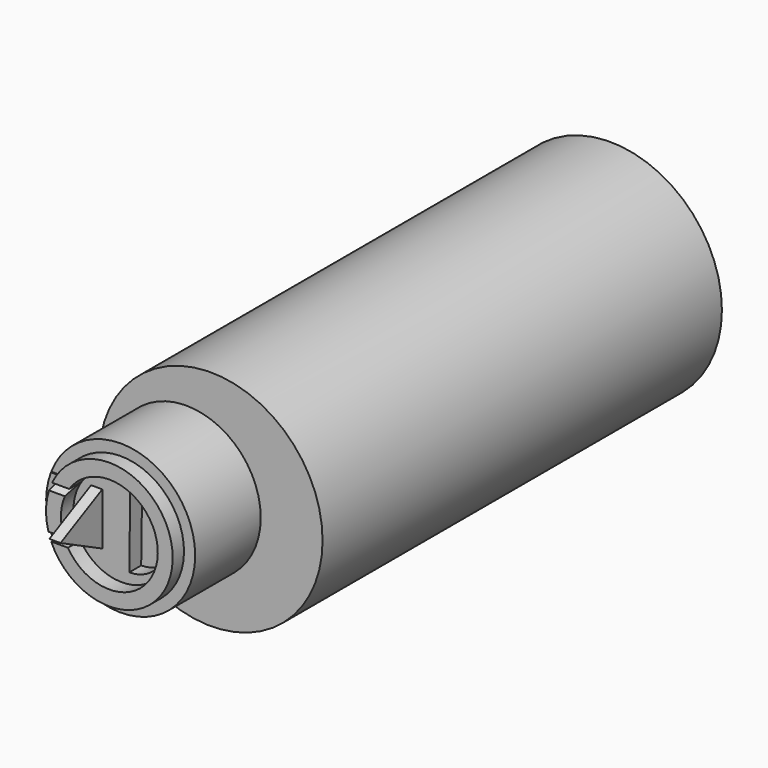
from build123d import *
from build123d import SkipClean  # not in build123d's __all__

# Parameters (mm, degrees)
F0_R      = 15
F1_DEPTH  = 67
F2_R      = 10
F3_DEPTH  = 11
F4_R      = 8.5
F5_DEPTH  = 1.9
F6_R      = 6.5
F7_DEPTH  = 2.1
F9_DEPTH  = 2
F10_W     = 1.5
F10_H     = 7
F11_DEPTH = 7
F13_DEPTH = 9.0692195411
F15_DEPTH = 25
F16_R     = 13.5
F17_DEPTH = 58.88


with BuildPart() as f1:
    # F0 (on Front) → F1 (new body)
    with BuildSketch(Plane.XZ):
        Circle(F0_R)
    extrude(amount=F1_DEPTH)

    # F2 (on face) → F3 (join)
    with BuildSketch(Plane.XZ.offset(67)):
        with Locations((-3.3, 0)):
            Circle(F2_R)
    extrude(amount=F3_DEPTH)

    # F4 (on face) → F5 (join)
    with BuildSketch(Plane.XZ.offset(78)):
        with Locations((-3.3, 0)):
            Circle(F4_R)
    extrude(amount=F5_DEPTH)

    # F6 (on face) → F7 (cut)
    with BuildSketch(Plane.XZ.offset(79.9)):
        with Locations((-3.3, 0)):
            Circle(F6_R)
    extrude(amount=-F7_DEPTH, mode=Mode.SUBTRACT)

    # F8 (on face) → F9 (cut)
    with BuildSketch(Plane.XZ.offset(77.8)):
        with BuildLine():
            ThreePointArc((-2.3067915896, -5), (1.2287423164, -3.5355339059), (2.6932084104, 0))
            ThreePointArc((2.6932084104, 0), (1.2757387706, 3.4879042731), (-2.1729820769, 4.9982091807))
            Line((-2.1729820769, 4.9982091807), (-2.3067915896, -5))
        make_face()
    extrude(amount=-F9_DEPTH, mode=Mode.SUBTRACT)

    # F10 (on face) → F11 (join)
    with BuildSketch(Plane.XZ.offset(77.8)):
        with Locations((-6.6817804589, 0.1302052614)):
            Rectangle(F10_W, F10_H)
    extrude(amount=F11_DEPTH)

    # F12 (on face) → F13 (cut, through all)
    with BuildSketch(Plane.YZ.offset(-5.9317804589)):
        Polygon((-77.8, -3.3697947386), (-84.8, 0.1302052614), (-84.8, -3.3697947386), align=None)
    with SkipClean():  # cleaning this boolean's faces spoils the solid; the shape is the same uncleaned
        extrude(amount=-F13_DEPTH, mode=Mode.SUBTRACT)

    # F14 (on face) → F15 (cut)
    with BuildSketch(Plane.YZ.offset(-5.9317804589)):
        Polygon((-84.8, 3.6302052614), (-84.8, 0.1302052614), (-77.8, 3.6302052614), align=None)
    extrude(amount=-F15_DEPTH, mode=Mode.SUBTRACT)

    # F16 (on face) → F17 (cut)
    with BuildSketch(Plane(origin=(0, 0, 0), x_dir=(-1, 0, 0), z_dir=(0, 1, 0))):
        Circle(F16_R)
    extrude(amount=-F17_DEPTH, mode=Mode.SUBTRACT)


solid = f1.part
